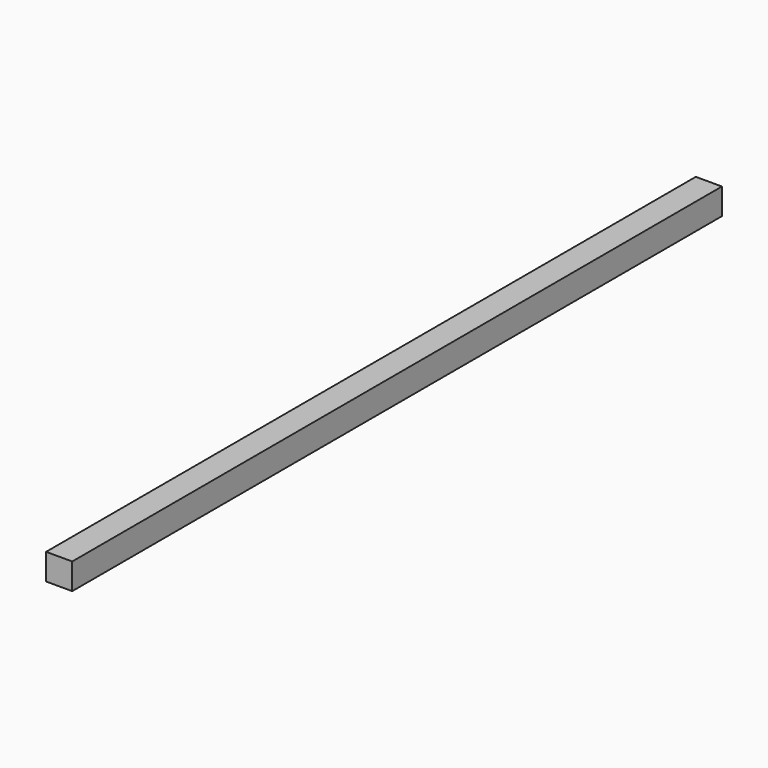
from build123d import *

# Parameters (mm, degrees)
F1_W     = 38.1
F1_H     = 38.1
F2_DEPTH = 1183.132


# Not quite as in the source:
# - a variable given as a bare number and used for a length is read in inches; the dataset says mm whatever the document's units were


with BuildPart() as f2:
    # F1 (on Front) → F2 (new body)
    with BuildSketch(Plane.XZ):
        Rectangle(F1_W, F1_H)
    extrude(amount=F2_DEPTH)


solid = f2.part
